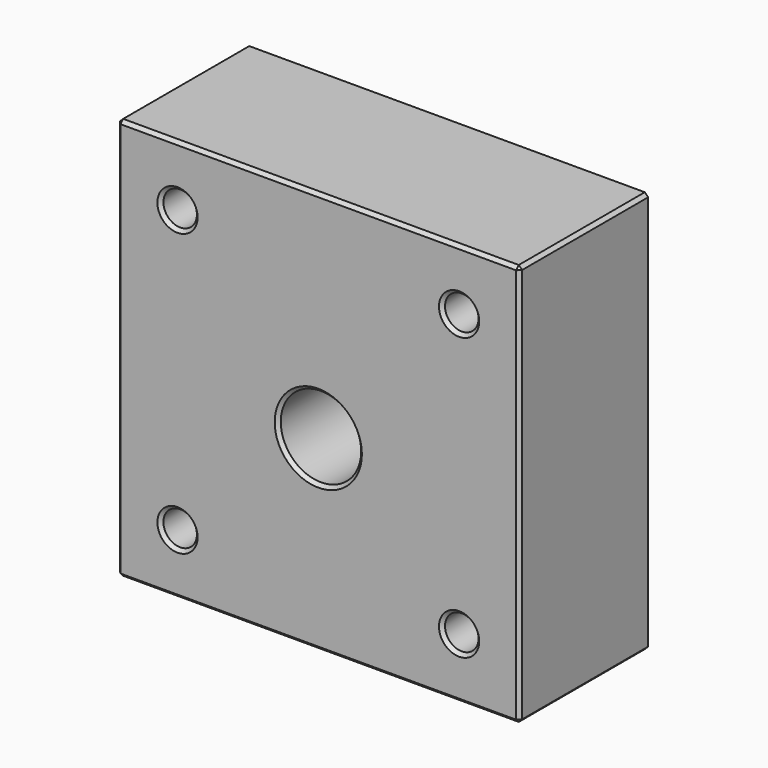
from build123d import *

# Parameters (mm, degrees)
F0_W     = 30
F0_H     = 30
F0_R     = 10
F0_R_2   = 3
F1_DEPTH = 12
F2_DEPTH = 3
F3_R     = 0.2
F4_R     = 12
F4_R_2   = 11
F5_DEPTH = 0.6
F6_R     = 0.49999
F4_R_3   = 1.25
F7_DEPTH = 25
F8_SIZE  = 0.25


# Not quite as in the source:
# - a fillet or chamfer is up to 0.001 mm smaller than in the source, because OpenCascade refuses the exact size


with BuildPart() as f1:
    # F0 (on Front) → F1 (new body)
    with BuildSketch(Plane.XZ):
        with Locations((15, -15)):
            Rectangle(F0_W, F0_H)
        with Locations((15, -15)):
            Circle(F0_R, mode=Mode.SUBTRACT)
        with Locations((15, -15)):
            Circle(F0_R)
        with Locations((15, -16.066)):
            Circle(F0_R_2, mode=Mode.SUBTRACT)
    extrude(amount=F1_DEPTH)

    # F0 (on Front) → F2 (cut)
    with BuildSketch(Plane.XZ):
        with Locations((15, -15)):
            Circle(F0_R)
        with Locations((15, -16.066)):
            Circle(F0_R_2, mode=Mode.SUBTRACT)
    extrude(amount=F2_DEPTH, mode=Mode.SUBTRACT)

    # F3
    f3_edges = [f1.edges().sort_by_distance(p)[0] for p in [
        (5, -3, -15),
    ]]
    fillet(f3_edges, radius=F3_R)

    # F4 (on face) → F5 (cut)
    with BuildSketch(Plane(origin=(0, 0, 0), x_dir=(-1, 0, 0), z_dir=(0, 1, 0))):
        with Locations((-15, -15)):
            Circle(F4_R)
        with Locations((-15, -15)):
            Circle(F4_R_2, mode=Mode.SUBTRACT)
    extrude(amount=-F5_DEPTH, mode=Mode.SUBTRACT)

    # F6 (radius 0.5 in the source; OpenCascade refuses exactly that, so slightly less here)
    f6_edges = [f1.edges().sort_by_distance(p)[0] for p in [
        (26, -0.6, -15),
        (27, -0.6, -15),
    ]]
    fillet(f6_edges, radius=F6_R)

    # F4 (on face) → F7 (cut)
    with BuildSketch(Plane(origin=(0, 0, 0), x_dir=(-1, 0, 0), z_dir=(0, 1, 0))):
        with Locations((-4.5, -4.5)):
            Circle(F4_R_3)
        with Locations((-25.5, -4.5)):
            Circle(F4_R_3)
        with Locations((-25.5, -25.5)):
            Circle(F4_R_3)
        with Locations((-4.5, -25.5)):
            Circle(F4_R_3)
    extrude(amount=-F7_DEPTH, mode=Mode.SUBTRACT)

    # F8
    f8_edges = [f1.edges().sort_by_distance(p)[0] for p in [
        (15, -12, 0),
        (30, -12, -15),
        (0, -12, -15),
        (15, -12, -30),
        (5.75, -12, -25.5),
        (26.75, -12, -25.5),
        (12, -12, -16.066),
        (5.75, -12, -4.5),
        (26.75, -12, -4.5),
        (30, -6, 0),
        (0, -6, 0),
        (30, -6, -30),
        (0, -6, -30),
        (5.75, 0, -4.5),
        (3.25, -6, -4.5),
        (26.75, 0, -25.5),
        (5.75, 0, -25.5),
        (3.25, -6, -25.5),
        (26.75, 0, -4.5),
    ]]
    chamfer(f8_edges, length=F8_SIZE)


solid = f1.part
